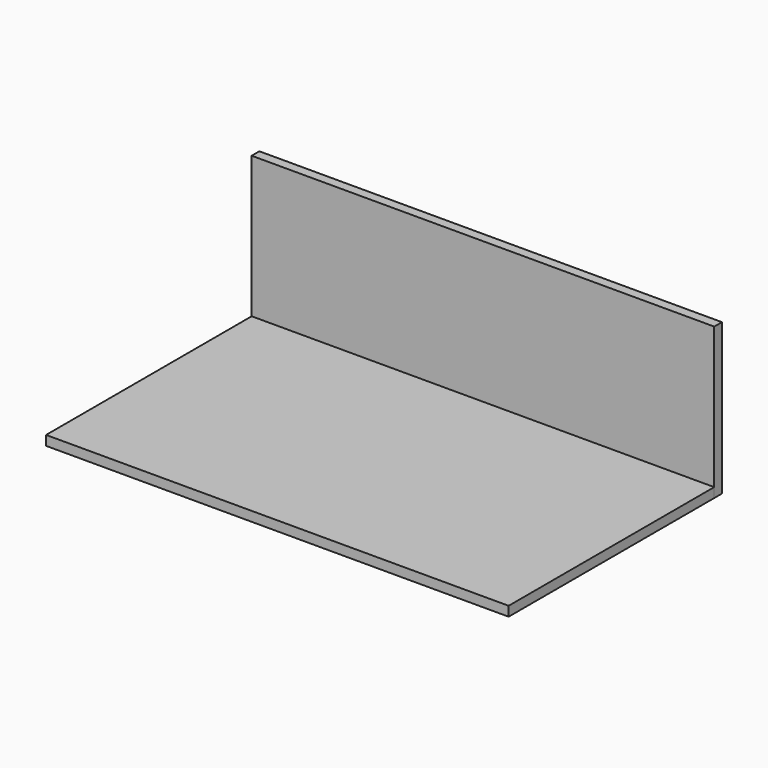
from build123d import *

# Parameters (mm, degrees)
F2_DEPTH = 3
F3_W     = 20.6222088363
F3_H     = 3
F3_W_2   = 39.1111204304
F3_W_3   = 39.1111154266
F3_W_4   = 11.022227565
F3_W_5   = 34.1333277417
F4_DEPTH = 44
F5_DEPTH = 3


with BuildPart() as f2:
    # F1 (on Top) → F2 (new body)
    with BuildSketch(Plane.XY):
        Polygon((0, 80), (0, 0), (144, 0), (144, 80), (123.3777911637, 80), (123.3777911637, 83), (84.2666707333, 83), (84.2666707333, 80), (50.1333429916, 80), (50.1333429916, 83), (11.022227565, 83), (11.022227565, 80), align=None)
    extrude(amount=F2_DEPTH)


with BuildPart() as f4:
    # F3 (on face) → F4 (new body)
    with BuildSketch(Plane.XY.offset(3)):
        with Locations((133.6888955819, 81.5)):
            Rectangle(F3_W, F3_H)
        with Locations((103.8222309485, 81.5)):
            Rectangle(F3_W_2, F3_H)
        with Locations((30.5777852783, 81.5)):
            Rectangle(F3_W_3, F3_H)
        with Locations((5.5111137825, 81.5)):
            Rectangle(F3_W_4, F3_H)
        with Locations((67.2000068624, 81.5)):
            Rectangle(F3_W_5, F3_H)
    extrude(amount=F4_DEPTH)

    # F3 (on face) → F5 (join)
    with BuildSketch(Plane.XY.offset(3)):
        with Locations((5.5111137825, 81.5)):
            Rectangle(F3_W_4, F3_H)
        with Locations((67.2000068624, 81.5)):
            Rectangle(F3_W_5, F3_H)
        with Locations((133.6888955819, 81.5)):
            Rectangle(F3_W, F3_H)
    extrude(amount=-F5_DEPTH)


solid = Compound([f2.part, f4.part])
